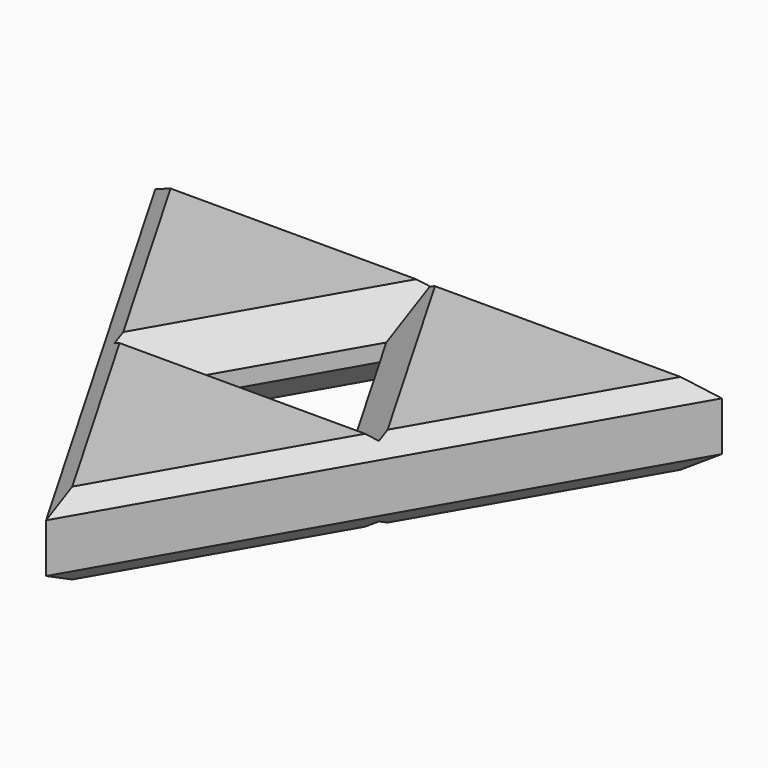
from build123d import *

# Parameters (mm, degrees)
F1_DEPTH    = 12.7
F2_SIZE     = 5.07999
F3_T1_DEPTH = 101.0523306034
F3_T3_DEPTH = 101.0523306034
F3_T5_DEPTH = 101.0523306034


# Not quite as in the source:
# - a fillet or chamfer that OpenCascade refuses, or shapes differently, is made with other operations: its cross-section is extruded or revolved along the edge and cut away or added
# - a fillet or chamfer is up to 0.001 mm smaller than in the source, because OpenCascade refuses the exact size


with BuildPart() as f1:
    # F0 (on Top) → F1 (new body)
    with BuildSketch(Plane.XY):
        Polygon((43.9940905122, 25.4), (0, 25.4), (2.9329393675, 20.32), (19.0641058886, -7.62), (21.9970452561, -12.7), align=None)
        Polygon((2.9329393675, 20.32), (0, 25.4), (-2.9329393675, 20.32), (0, 15.24), align=None)
        Polygon((-2.9329393675, 20.32), (0, 25.4), (-43.9940905122, 25.4), (-21.9970452561, -12.7), (-19.0641058886, -7.62), align=None)
        Polygon((19.0641058886, -7.62), (2.9329393675, 20.32), (0, 15.24), (13.1982271537, -7.62), align=None)
        Polygon((0, 15.24), (-2.9329393675, 20.32), (-19.0641058886, -7.62), (-13.1982271537, -7.62), align=None)
        Polygon((21.9970452561, -12.7), (19.0641058886, -7.62), (13.1982271537, -7.62), (16.1311665212, -12.7), align=None)
        Polygon((-13.1982271537, -7.62), (-19.0641058886, -7.62), (-21.9970452561, -12.7), (-16.1311665212, -12.7), align=None)
        Polygon((-16.1311665212, -12.7), (-21.9970452561, -12.7), (0, -50.8), (21.9970452561, -12.7), (16.1311665212, -12.7), align=None)
        Polygon((16.1311665212, -12.7), (13.1982271537, -7.62), (-13.1982271537, -7.62), (-16.1311665212, -12.7), align=None)
    extrude(amount=F1_DEPTH)

    # F2 (size 5.08 in the source; OpenCascade refuses exactly that, so slightly less here)
    f2_edges = [f1.edges().sort_by_distance(p)[0] for p in [
        (6.599114, 3.81, 12.7),
        (-6.599114, 3.81, 12.7),
        (0, -7.62, 12.7),
        (6.599114, 3.81, 0),
        (0, -7.62, 0),
        (-6.599114, 3.81, 0),
    ]]
    chamfer(f2_edges, length=F2_SIZE)

    # F3: chamfer of 2.54 on 6 edges, made by hand

    # F3_s2 → F3_t1 (cut)
    with BuildSketch(Plane(origin=(-25.2630826508, 43.7569427071, 0), x_dir=(0, 0, 1), z_dir=(0.5, -0.8660254038, 0))):
        with BuildLine():
            Line((12.771842049, 22.788157951), (10.088157951, 25.471842049))
            Line((10.088157951, 25.471842049), (10.088157951, 25.522642049))
            ThreePointArc((10.088157951, 25.522642049), (11.3940789755, 25.4508), (12.7, 25.4508))
            Line((12.7, 25.4508), (12.7508, 25.4))
            ThreePointArc((12.7508, 25.4), (12.7508, 24.0940789755), (12.822642049, 22.788157951))
            Line((12.822642049, 22.788157951), (12.771842049, 22.788157951))
        make_face()
        with BuildLine():
            Line((-0.071842049, 22.788157951), (2.611842049, 25.471842049))
            Line((2.611842049, 25.471842049), (2.611842049, 25.522642049))
            ThreePointArc((2.611842049, 25.522642049), (1.3059210245, 25.4508), (0, 25.4508))
            Line((0, 25.4508), (-0.0508, 25.4))
            ThreePointArc((-0.0508, 25.4), (-0.0508, 24.0940789755), (-0.122642049, 22.788157951))
            Line((-0.122642049, 22.788157951), (-0.071842049, 22.788157951))
        make_face()
    extrude(amount=F3_T1_DEPTH, mode=Mode.SUBTRACT)

    # F3_s4 → F3_t3 (cut)
    with BuildSketch(Plane(origin=(-25.2630826508, -43.7569427071, 0), x_dir=(0, 0, 1), z_dir=(0.5, 0.8660254038, 0))):
        with BuildLine():
            Line((12.771842049, 22.788157951), (10.088157951, 25.471842049))
            Line((10.088157951, 25.471842049), (10.088157951, 25.522642049))
            ThreePointArc((10.088157951, 25.522642049), (11.3940789755, 25.4508), (12.7, 25.4508))
            Line((12.7, 25.4508), (12.7508, 25.4))
            ThreePointArc((12.7508, 25.4), (12.7508, 24.0940789755), (12.822642049, 22.788157951))
            Line((12.822642049, 22.788157951), (12.771842049, 22.788157951))
        make_face()
        with BuildLine():
            Line((-0.071842049, 22.788157951), (2.611842049, 25.471842049))
            Line((2.611842049, 25.471842049), (2.611842049, 25.522642049))
            ThreePointArc((2.611842049, 25.522642049), (1.3059210245, 25.4508), (0, 25.4508))
            Line((0, 25.4508), (-0.0508, 25.4))
            ThreePointArc((-0.0508, 25.4), (-0.0508, 24.0940789755), (-0.122642049, 22.788157951))
            Line((-0.122642049, 22.788157951), (-0.071842049, 22.788157951))
        make_face()
    extrude(amount=F3_T3_DEPTH, mode=Mode.SUBTRACT)

    # F3_s6 → F3_t5 (cut)
    with BuildSketch(Plane.YZ.offset(-50.5261653017)):
        with BuildLine():
            Line((22.788157951, 12.771842049), (25.471842049, 10.088157951))
            Line((25.471842049, 10.088157951), (25.522642049, 10.088157951))
            ThreePointArc((25.522642049, 10.088157951), (25.4508, 11.3940789755), (25.4508, 12.7))
            Line((25.4508, 12.7), (25.4, 12.7508))
            ThreePointArc((25.4, 12.7508), (24.0940789755, 12.7508), (22.788157951, 12.822642049))
            Line((22.788157951, 12.822642049), (22.788157951, 12.771842049))
        make_face()
        with BuildLine():
            Line((22.788157951, -0.071842049), (25.471842049, 2.611842049))
            Line((25.471842049, 2.611842049), (25.522642049, 2.611842049))
            ThreePointArc((25.522642049, 2.611842049), (25.4508, 1.3059210245), (25.4508, 0))
            Line((25.4508, 0), (25.4, -0.0508))
            ThreePointArc((25.4, -0.0508), (24.0940789755, -0.0508), (22.788157951, -0.122642049))
            Line((22.788157951, -0.122642049), (22.788157951, -0.071842049))
        make_face()
    extrude(amount=F3_T5_DEPTH, mode=Mode.SUBTRACT)


solid = f1.part
